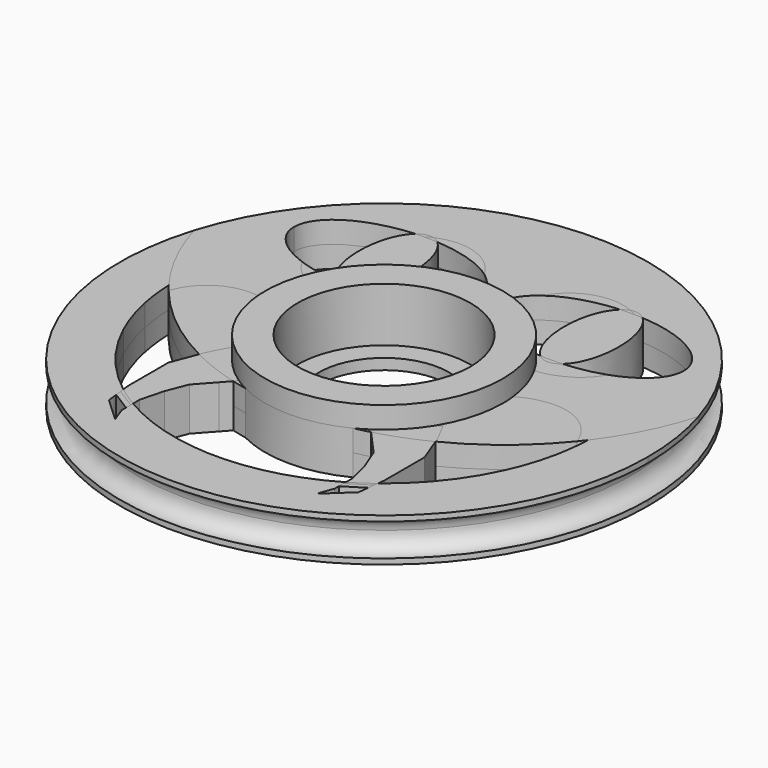
from build123d import *

# Parameters (mm, degrees)
F0_R      = 8
F1_DEPTH  = 2
F4_DEPTH  = 2
F5_DEPTH  = 2.5
F7_DEPTH  = 4
F8_DEPTH  = 25.4
F11_DEPTH = 4
F12_R     = 24.375
F12_R_2   = 8
F13_DEPTH = 4
F14_R     = 10.975
F15_DEPTH = 4
F16_DEPTH = 2
F17_R     = 7.975
F17_R_2   = 6
F18_DEPTH = 5
F19_DEPTH = 25
F9_R      = 1.5


with BuildPart() as f1:
    # F0 (on Top) → F1 (new body, symmetric)
    with BuildSketch(Plane.XY):
        with BuildLine():
            ThreePointArc((-23.2895913125, 7.1927436695), (-3.6370892728, -24.102120376), (24.375, 0))
            ThreePointArc((24.375, 0), (24.102120376, 3.6370892728), (23.2895913125, 7.1927436695))
            ThreePointArc((23.2895913125, 7.1927436695), (21.6842014138, 3.0935340882), (19.3641645477, -0.6478860777))
            ThreePointArc((19.3641645477, -0.6478860777), (19.2439090647, -2.2500197579), (18.9913269381, -3.8366816562))
            ThreePointArc((18.9913269381, -3.8366816562), (18.4267200032, -5.987204266), (17.6194511339, -8.0588812338))
            ThreePointArc((17.6194511339, -8.0588812338), (11.3883392632, -15.674704266), (2.2197416795, -19.2474250713))
            ThreePointArc((2.2197416795, -19.2474250713), (0, -19.375), (-2.2197416795, -19.2474250713))
            ThreePointArc((-2.2197416795, -19.2474250713), (-11.3883392632, -15.674704266), (-17.6194511339, -8.0588812338))
            ThreePointArc((-17.6194511339, -8.0588812338), (-18.4267200032, -5.987204266), (-18.9913269381, -3.8366816562))
            ThreePointArc((-18.9913269381, -3.8366816562), (-19.2439090647, -2.2500197579), (-19.3641645477, -0.6478860777))
            ThreePointArc((-19.3641645477, -0.6478860777), (-21.6842014138, 3.0935340882), (-23.2895913125, 7.1927436695))
        make_face()
        with BuildLine():
            ThreePointArc((19.3641645477, -0.6478860777), (21.6842014138, 3.0935340882), (23.2895913125, 7.1927436695))
            ThreePointArc((23.2895913125, 7.1927436695), (0, 24.375), (-23.2895913125, 7.1927436695))
            ThreePointArc((-23.2895913125, 7.1927436695), (-21.6842014138, 3.0935340882), (-19.3641645477, -0.6478860777))
            ThreePointArc((-19.3641645477, -0.6478860777), (-17.8673140003, 7.4933113784), (-13.1091613434, 14.2667625575))
            ThreePointArc((-13.1091613434, 14.2667625575), (-11.3883392632, 15.674704266), (-9.5175438596, 16.8762254038))
            ThreePointArc((-9.5175438596, 16.8762254038), (-4.878169917, 17.0192357628), (-2.1202405355, 13.2858635514))
            Line((-2.1202405355, 13.2858635514), (-2.0588370267, 12.8891487435))
            ThreePointArc((-2.0588370267, 12.8891487435), (-2.49086712, 9.9638648127), (-4.5, 7.7942286341))
            ThreePointArc((-4.5, 7.7942286341), (-5.2900672706, 7.2811529494), (-6.0221754572, 6.6883034293))
            ThreePointArc((-6.0221754572, 6.6883034293), (-8.5595086467, 2.7811529494), (-8.8033284066, -1.8712052174))
            ThreePointArc((-8.8033284066, -1.8712052174), (-8.5595086467, -2.7811529494), (-8.2219091188, -3.6606297877))
            ThreePointArc((-8.2219091188, -3.6606297877), (-5.2900672706, -7.2811529494), (-0.9407561694, -8.9506970583))
            ThreePointArc((-0.9407561694, -8.9506970583), (0, -9), (0.9407561694, -8.9506970583))
            ThreePointArc((0.9407561694, -8.9506970583), (5.2900672706, -7.2811529494), (8.2219091188, -3.6606297877))
            ThreePointArc((8.2219091188, -3.6606297877), (8.5595086467, -2.7811529494), (8.8033284066, -1.8712052174))
            ThreePointArc((8.8033284066, -1.8712052174), (8.5595086467, 2.7811529494), (6.0221754572, 6.6883034293))
            ThreePointArc((6.0221754572, 6.6883034293), (5.2900672706, 7.2811529494), (4.5, 7.7942286341))
            ThreePointArc((4.5, 7.7942286341), (2.49086712, 9.9638648127), (2.0588370267, 12.8891487435))
            Line((2.0588370267, 12.8891487435), (2.1202405355, 13.2858635514))
            ThreePointArc((2.1202405355, 13.2858635514), (4.878169917, 17.0192357628), (9.5175438596, 16.8762254038))
            ThreePointArc((9.5175438596, 16.8762254038), (11.3883392632, 15.674704266), (13.1091613434, 14.2667625575))
            ThreePointArc((13.1091613434, 14.2667625575), (17.8673140003, 7.4933113784), (19.3641645477, -0.6478860777))
        make_face()
        Circle(F0_R, mode=Mode.SUBTRACT)
        with BuildLine():
            ThreePointArc((18.8479292115, -1.3086045182), (19.1089027571, -0.9804766643), (19.3641645477, -0.6478860777))
            ThreePointArc((19.3641645477, -0.6478860777), (17.8673140003, 7.4933113784), (13.1091613434, 14.2667625575))
            ThreePointArc((13.1091613434, 14.2667625575), (14.6788176688, 9.8986483691), (11.9804167475, 6.1220261997))
            Line((11.9804167475, 6.1220261997), (11.6220932721, 5.941036375))
            ThreePointArc((11.6220932721, 5.941036375), (8.7064782868, 5.4479589625), (6.0221754572, 6.6883034293))
            ThreePointArc((6.0221754572, 6.6883034293), (8.5595086467, 2.7811529494), (8.8033284066, -1.8712052174))
            ThreePointArc((8.8033284066, -1.8712052174), (10.2459188284, 0.710048151), (12.8945245319, 2.0248956345))
            Line((12.8945245319, 2.0248956345), (13.2907974628, 2.0890890449))
            ThreePointArc((13.2907974628, 2.0890890449), (16.6985219199, 1.4192688869), (18.8479292115, -1.3086045182))
        make_face()
        with BuildLine():
            ThreePointArc((-13.1091613434, 14.2667625575), (-17.8673140003, 7.4933113784), (-19.3641645477, -0.6478860777))
            ThreePointArc((-19.3641645477, -0.6478860777), (-19.1089027571, -0.9804766643), (-18.8479292115, -1.3086045182))
            ThreePointArc((-18.8479292115, -1.3086045182), (-16.6985219199, 1.4192688869), (-13.2907974628, 2.0890890449))
            Line((-13.2907974628, 2.0890890449), (-12.8945245319, 2.0248956345))
            ThreePointArc((-12.8945245319, 2.0248956345), (-10.2459188284, 0.710048151), (-8.8033284066, -1.8712052174))
            ThreePointArc((-8.8033284066, -1.8712052174), (-8.5595086467, 2.7811529494), (-6.0221754572, 6.6883034293))
            ThreePointArc((-6.0221754572, 6.6883034293), (-8.7064782868, 5.4479589625), (-11.6220932721, 5.941036375))
            Line((-11.6220932721, 5.941036375), (-11.9804167475, 6.1220261997))
            ThreePointArc((-11.9804167475, 6.1220261997), (-14.6788176688, 9.8986483691), (-13.1091613434, 14.2667625575))
        make_face()
        with BuildLine():
            ThreePointArc((8.7647729915, -8.6608723715), (14.2873822439, -5.6444413083), (18.8479292115, -1.3086045182))
            ThreePointArc((18.8479292115, -1.3086045182), (16.6985219199, 1.4192688869), (13.2907974628, 2.0890890449))
            Line((13.2907974628, 2.0890890449), (12.8945245319, 2.0248956345))
            ThreePointArc((12.8945245319, 2.0248956345), (10.2459188284, 0.710048151), (8.8033284066, -1.8712052174))
            ThreePointArc((8.8033284066, -1.8712052174), (8.5595086467, -2.7811529494), (8.2219091188, -3.6606297877))
            ThreePointArc((8.2219091188, -3.6606297877), (7.8188457028, -6.2339793586), (8.7647729915, -8.6608723715))
        make_face()
        with BuildLine():
            ThreePointArc((-13.2907974628, 2.0890890449), (-16.6985219199, 1.4192688869), (-18.8479292115, -1.3086045182))
            ThreePointArc((-18.8479292115, -1.3086045182), (-14.2873822439, -5.6444413083), (-8.7647729915, -8.6608723715))
            ThreePointArc((-8.7647729915, -8.6608723715), (-7.8188457028, -6.2339793586), (-8.2219091188, -3.6606297877))
            ThreePointArc((-8.2219091188, -3.6606297877), (-8.5595086467, -2.7811529494), (-8.8033284066, -1.8712052174))
            ThreePointArc((-8.8033284066, -1.8712052174), (-10.2459188284, 0.710048151), (-12.8945245319, 2.0248956345))
            Line((-12.8945245319, 2.0248956345), (-13.2907974628, 2.0890890449))
        make_face()
        with BuildLine():
            ThreePointArc((4.4231441975, -9.8934299463), (6.6226950322, -9.3783739723), (8.7647729915, -8.6608723715))
            ThreePointArc((8.7647729915, -8.6608723715), (7.8188457028, -6.2339793586), (8.2219091188, -3.6606297877))
            ThreePointArc((8.2219091188, -3.6606297877), (5.2900672706, -7.2811529494), (0.9407561694, -8.9506970583))
            ThreePointArc((0.9407561694, -8.9506970583), (2.769941468, -9.097029975), (4.4231441975, -9.8934299463))
        make_face()
        with BuildLine():
            ThreePointArc((-8.2219091188, -3.6606297877), (-7.8188457028, -6.2339793586), (-8.7647729915, -8.6608723715))
            ThreePointArc((-8.7647729915, -8.6608723715), (-6.6226950322, -9.3783739723), (-4.4231441975, -9.8934299463))
            ThreePointArc((-4.4231441975, -9.8934299463), (-2.769941468, -9.097029975), (-0.9407561694, -8.9506970583))
            ThreePointArc((-0.9407561694, -8.9506970583), (-5.2900672706, -7.2811529494), (-8.2219091188, -3.6606297877))
        make_face()
        with BuildLine():
            ThreePointArc((-4.4231441975, -9.8934299463), (0, -10.300227657), (4.4231441975, -9.8934299463))
            ThreePointArc((4.4231441975, -9.8934299463), (2.769941468, -9.097029975), (0.9407561694, -8.9506970583))
            ThreePointArc((0.9407561694, -8.9506970583), (0, -9), (-0.9407561694, -8.9506970583))
            ThreePointArc((-0.9407561694, -8.9506970583), (-2.769941468, -9.097029975), (-4.4231441975, -9.8934299463))
        make_face()
    extrude(amount=F1_DEPTH, both=True)

    # F0 (on Top) → F4 (join, symmetric)
    with BuildSketch(Plane.XY):
        with BuildLine():
            ThreePointArc((19.3641645477, -0.6478860777), (21.6842014138, 3.0935340882), (23.2895913125, 7.1927436695))
            ThreePointArc((23.2895913125, 7.1927436695), (0, 24.375), (-23.2895913125, 7.1927436695))
            ThreePointArc((-23.2895913125, 7.1927436695), (-21.6842014138, 3.0935340882), (-19.3641645477, -0.6478860777))
            ThreePointArc((-19.3641645477, -0.6478860777), (-17.8673140003, 7.4933113784), (-13.1091613434, 14.2667625575))
            ThreePointArc((-13.1091613434, 14.2667625575), (-11.3883392632, 15.674704266), (-9.5175438596, 16.8762254038))
            ThreePointArc((-9.5175438596, 16.8762254038), (-4.878169917, 17.0192357628), (-2.1202405355, 13.2858635514))
            Line((-2.1202405355, 13.2858635514), (-2.0588370267, 12.8891487435))
            ThreePointArc((-2.0588370267, 12.8891487435), (-2.49086712, 9.9638648127), (-4.5, 7.7942286341))
            ThreePointArc((-4.5, 7.7942286341), (-5.2900672706, 7.2811529494), (-6.0221754572, 6.6883034293))
            ThreePointArc((-6.0221754572, 6.6883034293), (-8.5595086467, 2.7811529494), (-8.8033284066, -1.8712052174))
            ThreePointArc((-8.8033284066, -1.8712052174), (-8.5595086467, -2.7811529494), (-8.2219091188, -3.6606297877))
            ThreePointArc((-8.2219091188, -3.6606297877), (-5.2900672706, -7.2811529494), (-0.9407561694, -8.9506970583))
            ThreePointArc((-0.9407561694, -8.9506970583), (0, -9), (0.9407561694, -8.9506970583))
            ThreePointArc((0.9407561694, -8.9506970583), (5.2900672706, -7.2811529494), (8.2219091188, -3.6606297877))
            ThreePointArc((8.2219091188, -3.6606297877), (8.5595086467, -2.7811529494), (8.8033284066, -1.8712052174))
            ThreePointArc((8.8033284066, -1.8712052174), (8.5595086467, 2.7811529494), (6.0221754572, 6.6883034293))
            ThreePointArc((6.0221754572, 6.6883034293), (5.2900672706, 7.2811529494), (4.5, 7.7942286341))
            ThreePointArc((4.5, 7.7942286341), (2.49086712, 9.9638648127), (2.0588370267, 12.8891487435))
            Line((2.0588370267, 12.8891487435), (2.1202405355, 13.2858635514))
            ThreePointArc((2.1202405355, 13.2858635514), (4.878169917, 17.0192357628), (9.5175438596, 16.8762254038))
            ThreePointArc((9.5175438596, 16.8762254038), (11.3883392632, 15.674704266), (13.1091613434, 14.2667625575))
            ThreePointArc((13.1091613434, 14.2667625575), (17.8673140003, 7.4933113784), (19.3641645477, -0.6478860777))
        make_face()
        Circle(F0_R, mode=Mode.SUBTRACT)
        with BuildLine():
            ThreePointArc((-13.1091613434, 14.2667625575), (-17.8673140003, 7.4933113784), (-19.3641645477, -0.6478860777))
            ThreePointArc((-19.3641645477, -0.6478860777), (-19.1089027571, -0.9804766643), (-18.8479292115, -1.3086045182))
            ThreePointArc((-18.8479292115, -1.3086045182), (-16.6985219199, 1.4192688869), (-13.2907974628, 2.0890890449))
            Line((-13.2907974628, 2.0890890449), (-12.8945245319, 2.0248956345))
            ThreePointArc((-12.8945245319, 2.0248956345), (-10.2459188284, 0.710048151), (-8.8033284066, -1.8712052174))
            ThreePointArc((-8.8033284066, -1.8712052174), (-8.5595086467, 2.7811529494), (-6.0221754572, 6.6883034293))
            ThreePointArc((-6.0221754572, 6.6883034293), (-8.7064782868, 5.4479589625), (-11.6220932721, 5.941036375))
            Line((-11.6220932721, 5.941036375), (-11.9804167475, 6.1220261997))
            ThreePointArc((-11.9804167475, 6.1220261997), (-14.6788176688, 9.8986483691), (-13.1091613434, 14.2667625575))
        make_face()
        with BuildLine():
            ThreePointArc((18.8479292115, -1.3086045182), (19.1089027571, -0.9804766643), (19.3641645477, -0.6478860777))
            ThreePointArc((19.3641645477, -0.6478860777), (17.8673140003, 7.4933113784), (13.1091613434, 14.2667625575))
            ThreePointArc((13.1091613434, 14.2667625575), (14.6788176688, 9.8986483691), (11.9804167475, 6.1220261997))
            Line((11.9804167475, 6.1220261997), (11.6220932721, 5.941036375))
            ThreePointArc((11.6220932721, 5.941036375), (8.7064782868, 5.4479589625), (6.0221754572, 6.6883034293))
            ThreePointArc((6.0221754572, 6.6883034293), (8.5595086467, 2.7811529494), (8.8033284066, -1.8712052174))
            ThreePointArc((8.8033284066, -1.8712052174), (10.2459188284, 0.710048151), (12.8945245319, 2.0248956345))
            Line((12.8945245319, 2.0248956345), (13.2907974628, 2.0890890449))
            ThreePointArc((13.2907974628, 2.0890890449), (16.6985219199, 1.4192688869), (18.8479292115, -1.3086045182))
        make_face()
        with BuildLine():
            ThreePointArc((11.9804167475, 6.1220261997), (14.6788176688, 9.8986483691), (13.1091613434, 14.2667625575))
            ThreePointArc((13.1091613434, 14.2667625575), (11.3883392632, 15.674704266), (9.5175438596, 16.8762254038))
            ThreePointArc((9.5175438596, 16.8762254038), (4.878169917, 17.0192357628), (2.1202405355, 13.2858635514))
            Line((2.1202405355, 13.2858635514), (2.0588370267, 12.8891487435))
            ThreePointArc((2.0588370267, 12.8891487435), (2.49086712, 9.9638648127), (4.5, 7.7942286341))
            ThreePointArc((4.5, 7.7942286341), (5.2900672706, 7.2811529494), (6.0221754572, 6.6883034293))
            ThreePointArc((6.0221754572, 6.6883034293), (8.7064782868, 5.4479589625), (11.6220932721, 5.941036375))
            Line((11.6220932721, 5.941036375), (11.9804167475, 6.1220261997))
        make_face()
        with BuildLine():
            ThreePointArc((-9.5175438596, 16.8762254038), (-11.3883392632, 15.674704266), (-13.1091613434, 14.2667625575))
            ThreePointArc((-13.1091613434, 14.2667625575), (-14.6788176688, 9.8986483691), (-11.9804167475, 6.1220261997))
            Line((-11.9804167475, 6.1220261997), (-11.6220932721, 5.941036375))
            ThreePointArc((-11.6220932721, 5.941036375), (-8.7064782868, 5.4479589625), (-6.0221754572, 6.6883034293))
            ThreePointArc((-6.0221754572, 6.6883034293), (-5.2900672706, 7.2811529494), (-4.5, 7.7942286341))
            ThreePointArc((-4.5, 7.7942286341), (-2.49086712, 9.9638648127), (-2.0588370267, 12.8891487435))
            Line((-2.0588370267, 12.8891487435), (-2.1202405355, 13.2858635514))
            ThreePointArc((-2.1202405355, 13.2858635514), (-4.878169917, 17.0192357628), (-9.5175438596, 16.8762254038))
        make_face()
    extrude(amount=F4_DEPTH, both=True)

    # F3 (on Top) → F5 (cut, symmetric)
    with BuildSketch(Plane.XY):
        with BuildLine():
            add(Edge.make_bspline(
                [(-17.9980447446, 12.1077606454), (-17.9980447446, 4.0545161987), (-5.2139137907, 8.0811384221), (7.5702171632, 12.1077606454), (-5.2139137907, 16.1343828688), (-17.9980447446, 20.1610050922), (-17.9980447446, 12.1077606454)],
                knots=[0, 0, 0, 2.0943951024, 2.0943951024, 4.1887902048, 4.1887902048, 6.2831853072, 6.2831853072, 6.2831853072], degree=2, weights=[1, 0.5, 1, 0.5, 1, 0.5, 1]))
        make_face()
        with BuildLine():
            add(Edge.make_bspline(
                [(17.9980447446, 12.1077606454), (17.9980447446, 20.1610050922), (5.2139137907, 16.1343828688), (-7.5702171632, 12.1077606454), (5.2139137907, 8.0811384221), (17.9980447446, 4.0545161987), (17.9980447446, 12.1077606454)],
                knots=[0, 0, 0, 2.0943951024, 2.0943951024, 4.1887902048, 4.1887902048, 6.2831853072, 6.2831853072, 6.2831853072], degree=2, weights=[1, 0.5, 1, 0.5, 1, 0.5, 1]))
        make_face()
    extrude(amount=F5_DEPTH, both=True, mode=Mode.SUBTRACT)

    # F6 (on face) → F7 (join)
    with BuildSketch(Plane.XY.offset(2)):
        Polygon((-9.8284361884, -5.4746470414), (-10.7273682952, -7.2069889866), (-11.8337459862, -10.1112294942), (-11.8337459862, -13.2229160517), (-11.8337459862, -14.7441858426), (-11.4639383583, -15.9357867849), (-9.8284361884, -16.9569402933), (-9.8284361884, -15.9197114408), (-9.2752482742, -13.7761048973), (-8.5146138445, -11.839943938), (-7.0567625898, -10.2201098165), (-6.2590704715, -9.3337855723), (-5.6126550771, -7.9827224836), align=None)
        Polygon((-11.4639383583, -15.9357867849), (-11.8337459862, -14.7441858426), (-11.710150087, -15.7820603178), align=None)
        Polygon((-9.8284361884, -16.9569402933), (-11.4639383583, -15.9357867849), (-11.2114083022, -16.7494937778), (-10.9623600792, -16.9736372623), (-9.8284361884, -17.5216346979), align=None)
        Polygon((-11.2114083022, -16.7494937778), (-11.4639383583, -15.9357867849), (-11.710150087, -15.7820603178), (-11.6052494469, -16.6629446949), (-10.9623600792, -16.9736372623), align=None)
        Polygon((-10.9623600792, -16.9736372623), (-11.6052494469, -16.6629446949), (-11.5225771442, -17.3571705818), (-10.4232272133, -18.3850694448), (-9.3130944297, -19.4129701704), (-9.8284361884, -17.9941691458), align=None)
        Polygon((-9.8284361884, -17.5216346979), (-10.9623600792, -16.9736372623), (-9.8284361884, -17.9941691458), align=None)
        Polygon((9.8284361884, -5.4746470414), (5.6126550771, -7.9827224836), (6.2590704715, -9.3337855723), (7.0567625898, -10.2201098165), (8.5146138445, -11.839943938), (9.2752482742, -13.7761048973), (9.8284361884, -15.9197114408), (9.8284361884, -16.9569402933), (11.710150087, -15.7820603178), (11.8337459862, -14.7441858426), (11.8337459862, -13.2229160517), (11.8337459862, -10.1112294942), (10.7273682952, -7.2069889866), align=None)
        Polygon((11.6052494469, -16.6629446949), (11.710150087, -15.7820603178), (9.8284361884, -16.9569402933), (9.8284361884, -17.5216346979), (10.9623600792, -16.9736372623), align=None)
        Polygon((11.5225771442, -17.3571705818), (11.6052494469, -16.6629446949), (10.9623600792, -16.9736372623), (9.8284361884, -17.9941691458), (9.3130944297, -19.4129701704), (10.4232272133, -18.3850694448), align=None)
        Polygon((10.9623600792, -16.9736372623), (9.8284361884, -17.5216346979), (9.8284361884, -17.9941691458), align=None)
    extrude(amount=-F7_DEPTH)

    # F6 (on face) → F8 (cut)
    with BuildSketch(Plane.XY.offset(2)):
        Polygon((-11.4639383583, -15.9357867849), (-11.710150087, -15.7820603178), (-11.6052494469, -16.6629446949), (-10.9623600792, -16.9736372623), (-11.2114083022, -16.7494937778), align=None)
        Polygon((-9.8284361884, -16.9569402933), (-11.4639383583, -15.9357867849), (-11.2114083022, -16.7494937778), (-10.9623600792, -16.9736372623), (-9.8284361884, -17.5216346979), align=None)
        Polygon((-9.8284361884, -17.5216346979), (-10.9623600792, -16.9736372623), (-9.8284361884, -17.9941691458), align=None)
        Polygon((-10.9623600792, -16.9736372623), (-11.6052494469, -16.6629446949), (-11.5225771442, -17.3571705818), (-10.4232272133, -18.3850694448), (-9.3130944297, -19.4129701704), (-9.8284361884, -17.9941691458), align=None)
        Polygon((10.9623600792, -16.9736372623), (9.8284361884, -17.5216346979), (9.8284361884, -17.9941691458), align=None)
        Polygon((11.5225771442, -17.3571705818), (11.6052494469, -16.6629446949), (10.9623600792, -16.9736372623), (9.8284361884, -17.9941691458), (9.3130944297, -19.4129701704), (10.4232272133, -18.3850694448), align=None)
        Polygon((11.710150087, -15.7820603178), (9.8284361884, -16.9569402933), (9.8284361884, -17.5216346979), (10.9623600792, -16.9736372623), (11.6052494469, -16.6629446949), align=None)
    extrude(amount=-F8_DEPTH, mode=Mode.SUBTRACT)

    # F10 (on face) → F11 (join)
    with BuildSketch(Plane.XY.offset(2)):
        with BuildLine():
            add(Edge.make_bspline(
                [(-9.4752907753, 7.0734946632), (-5.0895715441, 7.0734946632), (-7.2824311597, 14.6248936366), (-9.4752907753, 22.17629261), (-11.6681503909, 14.6248936366), (-13.8610100065, 7.0734946632), (-9.4752907753, 7.0734946632)],
                knots=[0, 0, 0, 2.0943951024, 2.0943951024, 4.1887902048, 4.1887902048, 6.2831853072, 6.2831853072, 6.2831853072], degree=2, weights=[1, 0.5, 1, 0.5, 1, 0.5, 1]))
        make_face()
        with BuildLine():
            add(Edge.make_bspline(
                [(9.4752907753, 7.0734946632), (13.8610100065, 7.0734946632), (11.6681503909, 14.6248936366), (9.4752907753, 22.17629261), (7.2824311597, 14.6248936366), (5.0895715441, 7.0734946632), (9.4752907753, 7.0734946632)],
                knots=[0, 0, 0, 2.0943951024, 2.0943951024, 4.1887902048, 4.1887902048, 6.2831853072, 6.2831853072, 6.2831853072], degree=2, weights=[1, 0.5, 1, 0.5, 1, 0.5, 1]))
        make_face()
    extrude(amount=-F11_DEPTH)

    # F12 (on face) → F13 (join)
    with BuildSketch(Plane.XY.offset(2)):
        Circle(F12_R)
        Polygon((-11.6398399481, -16.3724771428), (-12.14378234, -16.0578321666), (-11.710150087, -15.7820603178), (-9.8284361884, -16.6970795977), (-9.0425019691, -17.9941691458), (-9.8284361884, -17.5034577911), (-9.8284361884, -17.9941691458), (-9.3130944297, -19.4129701704), (-10.4232272133, -18.3850694448), (-11.5225771442, -17.3571705818), align=None, mode=Mode.SUBTRACT)
        with BuildLine():
            ThreePointArc((-11.7554975618, -15.4012630026), (-17.2198686152, -8.8806953487), (-19.3641645477, -0.6478860777))
            ThreePointArc((-19.3641645477, -0.6478860777), (-15.5460720527, -4.6615721471), (-10.9167219416, -7.7040421489))
            Line((-10.9167219416, -7.7040421489), (-11.8337459862, -10.1112294942))
            Line((-11.8337459862, -10.1112294942), (-11.8337459862, -14.7441858426))
            Line((-11.8337459862, -14.7441858426), (-11.7554975618, -15.4012630026))
        make_face(mode=Mode.SUBTRACT)
        with BuildLine():
            ThreePointArc((9.8284361884, -16.6970795977), (0, -19.375), (-9.8284361884, -16.6970795977))
            Line((-9.8284361884, -16.6970795977), (-9.8284361884, -15.9197114408))
            Line((-9.8284361884, -15.9197114408), (-9.2752482742, -13.7761048973))
            Line((-9.2752482742, -13.7761048973), (-8.5146138445, -11.839943938))
            Line((-8.5146138445, -11.839943938), (-6.3639252273, -9.4502908129))
            ThreePointArc((-6.3639252273, -9.4502908129), (0, -10.300227657), (6.3639252273, -9.4502908129))
            Line((6.3639252273, -9.4502908129), (8.5146138445, -11.839943938))
            Line((8.5146138445, -11.839943938), (9.2752482742, -13.7761048973))
            Line((9.2752482742, -13.7761048973), (9.8284361884, -15.9197114408))
            Line((9.8284361884, -15.9197114408), (9.8284361884, -16.6970795977))
        make_face(mode=Mode.SUBTRACT)
        Polygon((9.0425019691, -17.9941691458), (9.8284361884, -16.6970795977), (11.710150087, -15.7820603178), (12.14378234, -16.0578321666), (11.6398399481, -16.3724771428), (11.5225771442, -17.3571705818), (10.4232272133, -18.3850694448), (9.3130944297, -19.4129701704), (9.8284361884, -17.9941691458), (9.8284361884, -17.5034577911), align=None, mode=Mode.SUBTRACT)
        with BuildLine():
            Line((11.8337459862, -10.1112294942), (10.9167219416, -7.7040421489))
            ThreePointArc((10.9167219416, -7.7040421489), (15.5460720527, -4.6615721471), (19.3641645477, -0.6478860777))
            ThreePointArc((19.3641645477, -0.6478860777), (17.2198686152, -8.8806953487), (11.7554975618, -15.4012630026))
            Line((11.7554975618, -15.4012630026), (11.8337459862, -14.7441858426))
            Line((11.8337459862, -14.7441858426), (11.8337459862, -10.1112294942))
        make_face(mode=Mode.SUBTRACT)
        with BuildLine():
            add(Edge.make_bspline(
                [(-10.4848667172, 7.490954143), (-10.0019134723, 7.0734946632), (-9.4752907753, 7.0734946632)],
                knots=[5.8341302481, 5.8341302481, 5.8341302481, 6.2831853072, 6.2831853072, 6.2831853072], degree=2, weights=[0.8315627921, 0.8927960014, 1]))
            add(Edge.make_bspline(
                [(-10.4848667172, 7.490954143), (-10.8927948171, 7.5175027363), (-11.2999446707, 7.5566938531), (-11.7058255012, 7.6087148125), (-12.1098622278, 7.673883337), (-12.5113924038, 7.7526496326), (-12.9096598316, 7.8456270549), (-13.4721348312, 7.9999116894), (-13.6397053879, 8.0488432823), (-13.8064233224, 8.1005983405), (-13.9721997516, 8.1552520532), (-14.1369330435, 8.2128879612), (-14.3005081036, 8.2735997921), (-14.6439857558, 8.4088290642), (-14.8235613835, 8.4841265751), (-15.0013490308, 8.5635372976), (-15.1771341052, 8.6472231307), (-15.3506578455, 8.735361894), (-15.5216142317, 8.8281528172), (-15.8659540867, 9.0283014507), (-16.0390080601, 9.1361308534), (-16.2084215228, 9.2495877242), (-16.3736771979, 9.3689469239), (-16.5341241834, 9.4944835747), (-16.688974313, 9.6264759472), (-16.9598676451, 9.8798517065), (-17.0779434893, 9.9990644767), (-17.1910095452, 10.1230101269), (-17.2984162483, 10.2517962685), (-17.3993956657, 10.3854617684), (-17.493090393, 10.523953406), (-17.6905491143, 10.8545026133), (-17.788534818, 11.0499919823), (-17.8703247447, 11.2529007332), (-17.9336955408, 11.462115655), (-17.9766777552, 11.675990113), (-17.9980451007, 11.8922321922), (-17.9980447446, 12.1077606454)],
                knots=[0.7810589954, 0.7810589954, 0.7810589954, 0.7810589954, 0.7810589954, 0.7810589954, 0.7810589954, 0.7810589954, 0.8462339891, 0.8462339891, 0.8462339891, 0.8462339891, 0.8462339891, 0.8462339891, 0.8740725759, 0.8740725759, 0.8740725759, 0.8740725759, 0.8740725759, 0.8740725759, 0.9051537664, 0.9051537664, 0.9051537664, 0.9051537664, 0.9051537664, 0.9051537664, 0.9377657574, 0.9377657574, 0.9377657574, 0.9377657574, 0.9377657574, 0.9377657574, 0.9647151576, 0.9647151576, 0.9647151576, 0.9647151576, 0.9647151576, 0.9647151576, 1, 1, 1, 1, 1, 1, 1, 1], degree=7))
            add(Edge.make_bspline(
                [(-17.9980447446, 12.1077606454), (-17.9980449154, 12.3059525922), (-17.9799774166, 12.5047102203), (-17.9436601691, 12.701686678), (-17.8899429753, 12.8950627241), (-17.8202515111, 13.0834652058), (-17.7362691284, 13.265901184), (-17.5763743211, 13.5571642314), (-17.5075616892, 13.6698065119), (-17.4337795972, 13.7795008943), (-17.3554755315, 13.8861747634), (-17.2730690675, 13.9898064511), (-17.186937499, 14.0904151447), (-16.9591801746, 14.3387759565), (-16.8128931147, 14.4823687593), (-16.6597096869, 14.6190496684), (-16.5006309467, 14.7490701354), (-16.3364871163, 14.8727074257), (-16.1679350944, 14.9902594447), (-15.8259209, 15.211911082), (-15.6526377323, 15.316176674), (-15.476095295, 15.4151140151), (-15.2967091798, 15.5089682646), (-15.1148262627, 15.5979592749), (-14.930729229, 15.6822887992), (-14.5800576575, 15.8327776441), (-14.4139280289, 15.8999050605), (-14.2464137173, 15.9636571353), (-14.0776573176, 16.0241463123), (-13.9077835288, 16.0814727031), (-13.736900169, 16.1357264994), (-13.1363031784, 16.3149388346), (-12.7019700403, 16.424208706), (-12.2633498786, 16.5161529645), (-11.8214941196, 16.5916301483), (-11.3773066078, 16.6512659416), (-10.9315532233, 16.6954960816), (-10.4848667456, 16.7245671234)],
                knots=[0, 0, 0, 0, 0, 0, 0, 0, 0.0341006764, 0.0341006764, 0.0341006764, 0.0341006764, 0.0341006764, 0.0341006764, 0.0564953949, 0.0564953949, 0.0564953949, 0.0564953949, 0.0564953949, 0.0564953949, 0.0910672296, 0.0910672296, 0.0910672296, 0.0910672296, 0.0910672296, 0.0910672296, 0.1250486814, 0.1250486814, 0.1250486814, 0.1250486814, 0.1250486814, 0.1250486814, 0.1551030463, 0.1551030463, 0.1551030463, 0.1551030463, 0.1551030463, 0.1551030463, 0.2301152173, 0.2301152173, 0.2301152173, 0.2301152173, 0.2301152173, 0.2301152173, 0.2301152173, 0.2301152173], degree=7))
            add(Edge.make_bspline(
                [(-8.465714785, 16.7245671061), (-9.4752907634, 17.5972335416), (-10.4848667456, 16.7245671234)],
                knots=[2.764360552, 2.764360552, 2.764360552, 3.518824747, 3.518824747, 3.518824747], degree=2, weights=[0.7824414352, 0.7175585655, 0.7824414338]))
            add(Edge.make_bspline(
                [(-8.465714785, 16.7245671061), (-8.0002738177, 16.6942754844), (-7.5360578395, 16.647538935), (-7.073796456, 16.5841064743), (-6.6143940282, 16.5035097716), (-6.158936102, 16.4050727551), (-5.7087041413, 16.287867067), (-5.2322455857, 16.1401934808), (-5.1992765387, 16.1298512637), (-5.1663441333, 16.1193958022), (-5.1334465654, 16.1088256645), (-5.1005838097, 16.0981399492), (-5.0677576198, 16.0873382853), (-4.7591965899, 15.9845907829), (-4.486153891, 15.8845366621), (-4.2162526232, 15.7758365436), (-3.9500828752, 15.6579985371), (-3.688411242, 15.5304735027), (-3.4322023248, 15.3926147635), (-2.9455912593, 15.1019971549), (-2.7147396632, 14.9504428961), (-2.490969252, 14.7881378178), (-2.2757357193, 14.6143049684), (-2.0710475932, 14.4282347468), (-1.8794649749, 14.2292963322), (-1.6272035052, 13.923693073), (-1.5534276066, 13.8279303489), (-1.4830917076, 13.7295864636), (-1.4165140331, 13.6286629903), (-1.354041499, 13.5251966282), (-1.2960376281, 13.4192669254), (-1.1641519753, 13.150711919), (-1.0960008329, 12.9852384905), (-1.0396868466, 12.8151294747), (-0.9964022796, 12.6411545422), (-0.9671468755, 12.4643352657), (-0.9525367011, 12.2859849992), (-0.9525366787, 11.991718648), (-0.9587306129, 11.8756579707), (-0.9711207298, 11.7600014586), (-0.9896049749, 11.6451293071), (-1.0139955535, 11.5313814405), (-1.0440373661, 11.4190598899), (-1.1351121594, 11.1343523113), (-1.2040465443, 10.9644385436), (-1.2850725535, 10.7996325192), (-1.3768387284, 10.6404820921), (-1.4780164598, 10.4872536113), (-1.5874361046, 10.3400053141), (-1.8867946818, 9.9773455212), (-2.0870783179, 9.7706956099), (-2.3014420637, 9.5779775405), (-2.5270315066, 9.3984716409), (-2.7616276935, 9.2313759505), (-3.003644369, 9.0758154082), (-3.5132356193, 8.7787220421), (-3.7812231167, 8.6384374497), (-4.0548516883, 8.5091401996), (-4.3330949168, 8.3901277891), (-4.615140562, 8.2808088235), (-4.9003664207, 8.1806564331), (-5.24845365, 8.0701397608), (-5.3091304368, 8.0512928889), (-5.3704645194, 8.0326613599), (-5.4324605958, 8.0142524909), (-5.4951553573, 7.9960641682), (-5.558513014, 7.9781161965), (-6.0190777183, 7.8507783059), (-6.420254098, 7.7564092076), (-6.825057405, 7.6764413503), (-7.2326689731, 7.6102817401), (-7.6423761905, 7.5574955705), (-8.0535646709, 7.5177775196), (-8.4657148263, 7.4909541491)],
                knots=[0.2785018769, 0.2785018769, 0.2785018769, 0.2785018769, 0.2785018769, 0.2785018769, 0.2785018769, 0.2785018769, 0.3567333289, 0.3567333289, 0.3567333289, 0.3567333289, 0.3567333289, 0.3567333289, 0.3625568396, 0.3625568396, 0.3625568396, 0.3625568396, 0.3625568396, 0.3625568396, 0.4114866164, 0.4114866164, 0.4114866164, 0.4114866164, 0.4114866164, 0.4114866164, 0.4579729123, 0.4579729123, 0.4579729123, 0.4579729123, 0.4579729123, 0.4579729123, 0.4783728688, 0.4783728688, 0.4783728688, 0.4783728688, 0.4783728688, 0.4783728688, 0.5085766716, 0.5085766716, 0.5085766716, 0.5085766716, 0.5085766716, 0.5085766716, 0.5282423976, 0.5282423976, 0.5282423976, 0.5282423976, 0.5282423976, 0.5282423976, 0.5591872741, 0.5591872741, 0.5591872741, 0.5591872741, 0.5591872741, 0.5591872741, 0.6076178522, 0.6076178522, 0.6076178522, 0.6076178522, 0.6076178522, 0.6076178522, 0.6584868188, 0.6584868188, 0.6584868188, 0.6584868188, 0.6584868188, 0.6584868188, 0.6691174168, 0.6691174168, 0.6691174168, 0.6691174168, 0.6691174168, 0.6691174168, 0.7350233151, 0.7350233151, 0.7350233151, 0.7350233151, 0.7350233151, 0.7350233151, 0.7350233151, 0.7350233151], degree=7))
            add(Edge.make_bspline(
                [(-9.4752907753, 7.0734946632), (-8.9486680743, 7.0734946632), (-8.4657148263, 7.4909541491)],
                knots=[0, 0, 0, 0.4490550622, 0.4490550622, 0.4490550622], degree=2, weights=[1, 0.8927960007, 0.8315627913]))
        make_face(mode=Mode.SUBTRACT)
        Circle(F12_R_2, mode=Mode.SUBTRACT)
        with BuildLine():
            add(Edge.make_bspline(
                [(10.4848667172, 16.7245671479), (9.4752907711, 17.5972335058), (8.4657148263, 16.7245671418)],
                knots=[2.7643605717, 2.7643605717, 2.7643605717, 3.5188247384, 3.5188247384, 3.5188247384], degree=2, weights=[0.7824414318, 0.7175585679, 0.7824414323]))
            add(Edge.make_bspline(
                [(10.4848667172, 16.7245671479), (10.8927948171, 16.6980185546), (11.2999446707, 16.6588274378), (11.7058255012, 16.6068064784), (12.1098622278, 16.5416379539), (12.5113924038, 16.4628716583), (12.9096598316, 16.369894236), (13.4721348312, 16.2156096015), (13.6397053879, 16.1666780086), (13.8064233224, 16.1149229504), (13.9721997516, 16.0602692377), (14.1369330435, 16.0026333297), (14.3005081036, 15.9419214988), (14.6439857558, 15.8066922267), (14.8235613835, 15.7313947158), (15.0013490308, 15.6519839933), (15.1771341052, 15.5682981602), (15.3506578455, 15.4801593969), (15.5216142317, 15.3873684737), (15.8659540867, 15.1872198402), (16.0390080601, 15.0793904375), (16.2084215228, 14.9659335667), (16.3736771979, 14.846574367), (16.5341241834, 14.7210377162), (16.688974313, 14.5890453437), (16.9598676451, 14.3356695844), (17.0779434893, 14.2164568142), (17.1910095452, 14.092511164), (17.2984162483, 13.9637250224), (17.3993956657, 13.8300595225), (17.493090393, 13.6915678849), (17.6905491143, 13.3610186776), (17.788534818, 13.1655293086), (17.8703247447, 12.9626205577), (17.9336955408, 12.7534056359), (17.9766777552, 12.5395311779), (17.9980451007, 12.3232890987), (17.9980447446, 12.1077606454)],
                knots=[0.7810589954, 0.7810589954, 0.7810589954, 0.7810589954, 0.7810589954, 0.7810589954, 0.7810589954, 0.7810589954, 0.8462339891, 0.8462339891, 0.8462339891, 0.8462339891, 0.8462339891, 0.8462339891, 0.8740725759, 0.8740725759, 0.8740725759, 0.8740725759, 0.8740725759, 0.8740725759, 0.9051537664, 0.9051537664, 0.9051537664, 0.9051537664, 0.9051537664, 0.9051537664, 0.9377657574, 0.9377657574, 0.9377657574, 0.9377657574, 0.9377657574, 0.9377657574, 0.9647151576, 0.9647151576, 0.9647151576, 0.9647151576, 0.9647151576, 0.9647151576, 1, 1, 1, 1, 1, 1, 1, 1], degree=7))
            add(Edge.make_bspline(
                [(17.9980447446, 12.1077606454), (17.9980449154, 11.9095686987), (17.9799774166, 11.7108110706), (17.9436601691, 11.5138346129), (17.8899429753, 11.3204585668), (17.8202515111, 11.1320560851), (17.7362691284, 10.9496201069), (17.5763743211, 10.6583570595), (17.5075616892, 10.545714779), (17.4337795972, 10.4360203966), (17.3554755315, 10.3293465275), (17.2730690675, 10.2257148398), (17.186937499, 10.1251061462), (16.9591801746, 9.8767453344), (16.8128931147, 9.7331525316), (16.6597096869, 9.5964716225), (16.5006309467, 9.4664511555), (16.3364871163, 9.3428138652), (16.1679350944, 9.2252618462), (15.8259209, 9.0036102089), (15.6526377323, 8.8993446169), (15.476095295, 8.8004072758), (15.2967091798, 8.7065530263), (15.1148262627, 8.617562016), (14.930729229, 8.5332324917), (14.5800576575, 8.3827436468), (14.4139280289, 8.3156162304), (14.2464137173, 8.2518641556), (14.0776573176, 8.1913749786), (13.9077835288, 8.1340485878), (13.736900169, 8.0797947915), (13.1363031784, 7.9005824563), (12.7019700403, 7.7913125849), (12.2633498786, 7.6993683264), (11.8214941196, 7.6238911426), (11.3773066078, 7.5642553493), (10.9315532233, 7.5200252093), (10.4848667456, 7.4909541675)],
                knots=[0, 0, 0, 0, 0, 0, 0, 0, 0.0341006764, 0.0341006764, 0.0341006764, 0.0341006764, 0.0341006764, 0.0341006764, 0.0564953949, 0.0564953949, 0.0564953949, 0.0564953949, 0.0564953949, 0.0564953949, 0.0910672296, 0.0910672296, 0.0910672296, 0.0910672296, 0.0910672296, 0.0910672296, 0.1250486814, 0.1250486814, 0.1250486814, 0.1250486814, 0.1250486814, 0.1250486814, 0.1551030463, 0.1551030463, 0.1551030463, 0.1551030463, 0.1551030463, 0.1551030463, 0.2301152173, 0.2301152173, 0.2301152173, 0.2301152173, 0.2301152173, 0.2301152173, 0.2301152173, 0.2301152173], degree=7))
            add(Edge.make_bspline(
                [(9.4752907753, 7.0734946632), (10.0019134884, 7.0734946632), (10.4848667456, 7.4909541675)],
                knots=[0, 0, 0, 0.4490550714, 0.4490550714, 0.4490550714], degree=2, weights=[1, 0.8927959985, 0.8315627888]))
            add(Edge.make_bspline(
                [(8.465714785, 7.4909541848), (8.9486680508, 7.0734946632), (9.4752907753, 7.0734946632)],
                knots=[5.8341302271, 5.8341302271, 5.8341302271, 6.2831853072, 6.2831853072, 6.2831853072], degree=2, weights=[0.8315627864, 0.8927959964, 1]))
            add(Edge.make_bspline(
                [(8.465714785, 7.4909541848), (8.0002738177, 7.5212458065), (7.5360578395, 7.5679823559), (7.073796456, 7.6314148166), (6.6143940282, 7.7120115193), (6.158936102, 7.8104485358), (5.7087041413, 7.9276542239), (5.2322455857, 8.0753278101), (5.1992765387, 8.0856700272), (5.1663441333, 8.0961254887), (5.1334465654, 8.1066956264), (5.1005838097, 8.1173813417), (5.0677576198, 8.1281830056), (4.7591965899, 8.230930508), (4.486153891, 8.3309846288), (4.2162526232, 8.4396847473), (3.9500828752, 8.5575227538), (3.688411242, 8.6850477882), (3.4322023248, 8.8229065274), (2.9455912593, 9.113524136), (2.7147396632, 9.2650783948), (2.490969252, 9.4273834731), (2.2757357193, 9.6012163225), (2.0710475932, 9.7872865441), (1.8794649749, 9.9862249587), (1.6272035052, 10.2918282179), (1.5534276066, 10.387590942), (1.4830917076, 10.4859348273), (1.4165140331, 10.5868583006), (1.354041499, 10.6903246627), (1.2960376281, 10.7962543655), (1.1641519753, 11.0648093719), (1.0960008329, 11.2302828004), (1.0396868466, 11.4003918162), (0.9964022796, 11.5743667486), (0.9671468755, 11.7511860252), (0.9525367011, 11.9295362917), (0.9525366787, 12.2238026429), (0.9587306129, 12.3398633202), (0.9711207298, 12.4555198323), (0.9896049749, 12.5703919838), (1.0139955535, 12.6841398504), (1.0440373661, 12.796461401), (1.1351121594, 13.0811689796), (1.2040465442, 13.2510827473), (1.2850725535, 13.4158887717), (1.3768387284, 13.5750391988), (1.4780164598, 13.7282676796), (1.5874361046, 13.8755159768), (1.8867946818, 14.2381757697), (2.0870783179, 14.444825681), (2.3014420637, 14.6375437504), (2.5270315066, 14.81704965), (2.7616276935, 14.9841453404), (3.003644369, 15.1397058827), (3.5132356193, 15.4367992488), (3.7812231167, 15.5770838412), (4.0548516883, 15.7063810913), (4.3330949168, 15.8253935018), (4.615140562, 15.9347124674), (4.9003664207, 16.0348648578), (5.24845365, 16.1453815301), (5.3091304368, 16.164228402), (5.3704645194, 16.182859931), (5.4324605958, 16.2012688), (5.4951553573, 16.2194571227), (5.558513014, 16.2374050944), (6.0190777183, 16.364742985), (6.420254098, 16.4591120833), (6.825057405, 16.5390799406), (7.2326689731, 16.6052395508), (7.6423761905, 16.6580257204), (8.0535646709, 16.6977437713), (8.4657148263, 16.7245671418)],
                knots=[0.2785018769, 0.2785018769, 0.2785018769, 0.2785018769, 0.2785018769, 0.2785018769, 0.2785018769, 0.2785018769, 0.3567333289, 0.3567333289, 0.3567333289, 0.3567333289, 0.3567333289, 0.3567333289, 0.3625568396, 0.3625568396, 0.3625568396, 0.3625568396, 0.3625568396, 0.3625568396, 0.4114866164, 0.4114866164, 0.4114866164, 0.4114866164, 0.4114866164, 0.4114866164, 0.4579729123, 0.4579729123, 0.4579729123, 0.4579729123, 0.4579729123, 0.4579729123, 0.4783728688, 0.4783728688, 0.4783728688, 0.4783728688, 0.4783728688, 0.4783728688, 0.5085766716, 0.5085766716, 0.5085766716, 0.5085766716, 0.5085766716, 0.5085766716, 0.5282423976, 0.5282423976, 0.5282423976, 0.5282423976, 0.5282423976, 0.5282423976, 0.5591872741, 0.5591872741, 0.5591872741, 0.5591872741, 0.5591872741, 0.5591872741, 0.6076178522, 0.6076178522, 0.6076178522, 0.6076178522, 0.6076178522, 0.6076178522, 0.6584868188, 0.6584868188, 0.6584868188, 0.6584868188, 0.6584868188, 0.6584868188, 0.6691174168, 0.6691174168, 0.6691174168, 0.6691174168, 0.6691174168, 0.6691174168, 0.7350233151, 0.7350233151, 0.7350233151, 0.7350233151, 0.7350233151, 0.7350233151, 0.7350233151, 0.7350233151], degree=7))
        make_face(mode=Mode.SUBTRACT)
        Polygon((-11.710150087, -15.7820603178), (-12.14378234, -16.0578321666), (-9.0425019691, -17.9941691458), (-9.8284361884, -16.6970795977), align=None)
        Polygon((9.0425019691, -17.9941691458), (12.14378234, -16.0578321666), (11.710150087, -15.7820603178), (9.8284361884, -16.6970795977), align=None)
    extrude(amount=-F13_DEPTH)

    # F14 (on face) → F15 (join)
    with BuildSketch(Plane.XY.offset(2)):
        Circle(F14_R)
    extrude(amount=-F15_DEPTH)

    # F14 (on face) → F16 (join)
    with BuildSketch(Plane.XY.offset(2)):
        Circle(F14_R)
    extrude(amount=F16_DEPTH)

    # F17 (on face) → F18 (cut)
    with BuildSketch(Plane.XY.offset(4)):
        Circle(F17_R)
        Circle(F17_R_2, mode=Mode.SUBTRACT)
        Circle(F17_R_2)
    extrude(amount=-F18_DEPTH, mode=Mode.SUBTRACT)

    # F17 (on face) → F19 (cut)
    with BuildSketch(Plane.XY.offset(4)):
        Circle(F17_R_2)
    extrude(amount=-F19_DEPTH, mode=Mode.SUBTRACT)

    # F9 (on Front) → F20 (revolve, cut)
    with BuildSketch(Plane.XZ):
        with Locations((-24.3750531226, 0)):
            Circle(F9_R)
    revolve(axis=Axis((0, 0, -0.5204055458), (0, 0, -1)), mode=Mode.SUBTRACT)


solid = f1.part
